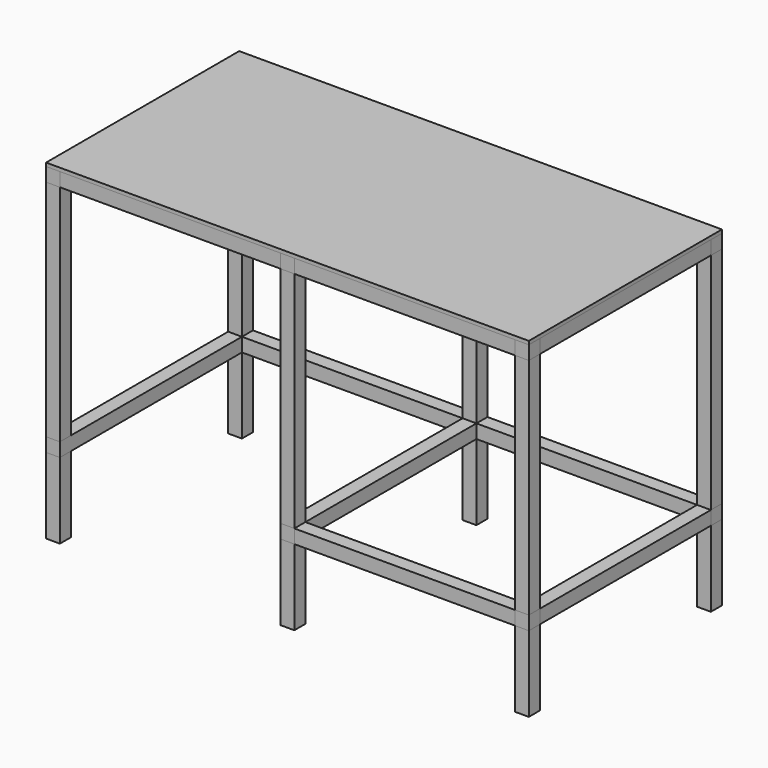
from build123d import *

# Parameters (mm, degrees)
F0_W     = 40
F0_H     = 40
F1_DEPTH = 950
F2_W     = 40
F2_H     = 40
F3_DEPTH = 720
F2_W_2   = 700
F2_H_2   = 10
F4_DEPTH = 1400
F5_W     = 40
F5_H     = 40
F6_DEPTH = 700
F7_W     = 40
F7_H     = 40
F8_DEPTH = 1400


# Not quite as in the source:
# - a feature names something its author has since deleted; it is built from what else it names


with BuildPart() as f1:
    # F0 (on Top) → F1 (new body)
    with BuildSketch(Plane.XY):
        with Locations((-1380.0028958117, -19.9983263365)):
            Rectangle(F0_W, F0_H)
    extrude(amount=F1_DEPTH)


with BuildPart() as f1b:
    # F0 (on Top) → F1, piece 2 (new body)
    with BuildSketch(Plane.XY):
        with Locations((-700.0028958117, -19.9983263365)):
            Rectangle(F0_W, F0_H)
    extrude(amount=F1_DEPTH)


with BuildPart() as f1c:
    # F0 (on Top) → F1, piece 3 (new body)
    with BuildSketch(Plane.XY):
        with Locations((-1380.0028958117, -679.9983263365)):
            Rectangle(F0_W, F0_H)
    extrude(amount=F1_DEPTH)


with BuildPart() as f1d:
    # F0 (on Top) → F1, piece 4 (new body)
    with BuildSketch(Plane.XY):
        with Locations((-700.0028958117, -679.9983263365)):
            Rectangle(F0_W, F0_H)
    extrude(amount=F1_DEPTH)


with BuildPart() as f1e:
    # F0 (on Top) → F1, piece 5 (new body)
    with BuildSketch(Plane.XY):
        with Locations((-20.0028958117, -679.9983263365)):
            Rectangle(F0_W, F0_H)
    extrude(amount=F1_DEPTH)


with BuildPart() as f1f:
    # F0 (on Top) → F1, piece 6 (new body)
    with BuildSketch(Plane.XY):
        with Locations((-20.0028958117, -19.9983263365)):
            Rectangle(F0_W, F0_H)
    extrude(amount=F1_DEPTH)


with BuildPart() as f3:
    # F2 (on Right) → F3 (new body)
    with BuildSketch(Plane.YZ):
        with Locations((-679.9983263365, 240)):
            Rectangle(F2_W, F2_H)
    extrude(amount=-F3_DEPTH)


with BuildPart() as f4:
    # F2 (on Right) → F4 (new body)
    with BuildSketch(Plane.YZ):
        with Locations((-349.9983263365, 955)):
            Rectangle(F2_W_2, F2_H_2)
    extrude(amount=-F4_DEPTH)


with BuildPart() as f4b:
    # F2 (on Right) → F4, piece 2 (new body)
    with BuildSketch(Plane.YZ):
        with Locations((-19.9983263365, 240)):
            Rectangle(F2_W, F2_H)
    extrude(amount=-F4_DEPTH)


with BuildPart() as f6:
    # F5 (on Front) → F6 (new body)
    with BuildSketch(Plane.XZ):
        with Locations((-20.0028958117, 240)):
            Rectangle(F5_W, F5_H)
    extrude(amount=F6_DEPTH)


with BuildPart() as f6b:
    # F5 (on Front) → F6, piece 2 (new body)
    with BuildSketch(Plane.XZ):
        with Locations((-700.0028958117, 240)):
            Rectangle(F5_W, F5_H)
    extrude(amount=F6_DEPTH)


with BuildPart() as f6c:
    # F5 (on Front) → F6, piece 3 (new body)
    with BuildSketch(Plane.XZ):
        with Locations((-1380.0028958117, 240)):
            Rectangle(F5_W, F5_H)
    extrude(amount=F6_DEPTH)


with BuildPart() as f6d:
    # F5 (on Front) → F6, piece 4 (new body)
    with BuildSketch(Plane.XZ):
        with Locations((-20.0028958117, 930)):
            Rectangle(F5_W, F5_H)
    extrude(amount=F6_DEPTH)


with BuildPart() as f6e:
    # F5 (on Front) → F6, piece 5 (new body)
    with BuildSketch(Plane.XZ):
        with Locations((-700.0028958117, 930)):
            Rectangle(F5_W, F5_H)
    extrude(amount=F6_DEPTH)


with BuildPart() as f6f:
    # F5 (on Front) → F6, piece 6 (new body)
    with BuildSketch(Plane.XZ):
        with Locations((-1380.0028958117, 930)):
            Rectangle(F5_W, F5_H)
    extrude(amount=F6_DEPTH)


with BuildPart() as f8:
    # F7 (on Right) → F8 (new body)
    with BuildSketch(Plane.YZ):
        with Locations((-679.9983263365, 930)):
            Rectangle(F7_W, F7_H)
    extrude(amount=-F8_DEPTH)


with BuildPart() as f8b:
    # F7 (on Right) → F8, piece 2 (new body)
    with BuildSketch(Plane.YZ):
        with Locations((-19.9983263365, 930)):
            Rectangle(F7_W, F7_H)
    extrude(amount=-F8_DEPTH)


solid = Compound([f1.part, f1b.part, f1c.part, f1d.part, f1e.part, f1f.part, f3.part, f4.part, f4b.part, f6.part, f6b.part, f6c.part, f6d.part, f6e.part, f6f.part, f8.part, f8b.part])
